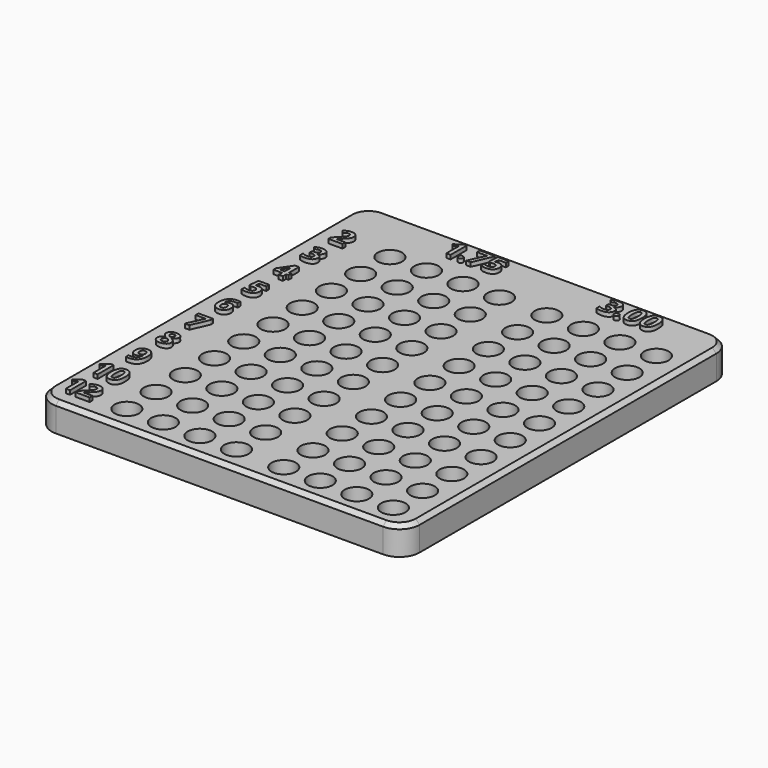
from build123d import *

# Parameters (mm, degrees)
F0_W         = 90.6357094646
F0_H         = 101.3200525194
F0_R         = 3
F1_DEPTH     = 7
F2_TEXT_SIZE = 6.9444444444
F3_DEPTH     = 1
F4_R         = 5
F5_SIZE      = 1


# Not quite as in the source:
# - Text() gives the source's letters only with a copy of the font that has no kerning and outlines rounded to 1/6400 em; it was checked with that copy


with BuildPart() as f1:
    # F0 (on Top) → F1 (new body)
    with BuildSketch(Plane.XY):
        with Locations((-1.2712031603, -23.1389431283)):
            Rectangle(F0_W, F0_H)
        with Locations((-28.8994200528, -67.7876200386)):
            Circle(F0_R, mode=Mode.SUBTRACT)
        with Locations((-28.8994200528, -58.7876200386)):
            Circle(F0_R, mode=Mode.SUBTRACT)
        with Locations((-28.8994200528, -49.7876200386)):
            Circle(F0_R, mode=Mode.SUBTRACT)
        with Locations((-19.8994200528, -67.7876200386)):
            Circle(F0_R, mode=Mode.SUBTRACT)
        with Locations((-10.8994200528, -67.7876200386)):
            Circle(F0_R, mode=Mode.SUBTRACT)
        with Locations((-1.8994200528, -67.7876200386)):
            Circle(F0_R, mode=Mode.SUBTRACT)
        with Locations((-19.8994200528, -58.7876200386)):
            Circle(F0_R, mode=Mode.SUBTRACT)
        with Locations((-19.8994200528, -49.7876200386)):
            Circle(F0_R, mode=Mode.SUBTRACT)
        with Locations((-10.8994200528, -58.7876200386)):
            Circle(F0_R, mode=Mode.SUBTRACT)
        with Locations((-1.8994200528, -58.7876200386)):
            Circle(F0_R, mode=Mode.SUBTRACT)
        with Locations((-10.8994200528, -49.7876200386)):
            Circle(F0_R, mode=Mode.SUBTRACT)
        with Locations((-1.8994200528, -49.7876200386)):
            Circle(F0_R, mode=Mode.SUBTRACT)
        with Locations((-28.8994200528, -40.7876200386)):
            Circle(F0_R, mode=Mode.SUBTRACT)
        with Locations((-28.8994200528, -31.7876200386)):
            Circle(F0_R, mode=Mode.SUBTRACT)
        with Locations((-19.8994200528, -40.7876200386)):
            Circle(F0_R, mode=Mode.SUBTRACT)
        with Locations((-10.8994200528, -40.7876200386)):
            Circle(F0_R, mode=Mode.SUBTRACT)
        with Locations((-1.8994200528, -40.7876200386)):
            Circle(F0_R, mode=Mode.SUBTRACT)
        with Locations((-19.8994200528, -31.7876200386)):
            Circle(F0_R, mode=Mode.SUBTRACT)
        with Locations((-10.8994200528, -31.7876200386)):
            Circle(F0_R, mode=Mode.SUBTRACT)
        with Locations((-1.8994200528, -31.7876200386)):
            Circle(F0_R, mode=Mode.SUBTRACT)
        with Locations((9.8412055522, -67.8979342282)):
            Circle(F0_R, mode=Mode.SUBTRACT)
        with Locations((18.8412055522, -67.8979342282)):
            Circle(F0_R, mode=Mode.SUBTRACT)
        with Locations((9.8412055522, -58.8979342282)):
            Circle(F0_R, mode=Mode.SUBTRACT)
        with Locations((9.8412055522, -49.8979342282)):
            Circle(F0_R, mode=Mode.SUBTRACT)
        with Locations((18.8412055522, -58.8979342282)):
            Circle(F0_R, mode=Mode.SUBTRACT)
        with Locations((18.8412055522, -49.8979342282)):
            Circle(F0_R, mode=Mode.SUBTRACT)
        with Locations((27.8412055522, -67.8979342282)):
            Circle(F0_R, mode=Mode.SUBTRACT)
        with Locations((36.8412055522, -67.8979342282)):
            Circle(F0_R, mode=Mode.SUBTRACT)
        with Locations((27.8412055522, -58.8979342282)):
            Circle(F0_R, mode=Mode.SUBTRACT)
        with Locations((27.8412055522, -49.8979342282)):
            Circle(F0_R, mode=Mode.SUBTRACT)
        with Locations((36.8412055522, -58.8979342282)):
            Circle(F0_R, mode=Mode.SUBTRACT)
        with Locations((36.8412055522, -49.8979342282)):
            Circle(F0_R, mode=Mode.SUBTRACT)
        with Locations((9.8412055522, -40.8979342282)):
            Circle(F0_R, mode=Mode.SUBTRACT)
        with Locations((18.8412055522, -40.8979342282)):
            Circle(F0_R, mode=Mode.SUBTRACT)
        with Locations((9.8412055522, -31.8979342282)):
            Circle(F0_R, mode=Mode.SUBTRACT)
        with Locations((18.8412055522, -31.8979342282)):
            Circle(F0_R, mode=Mode.SUBTRACT)
        with Locations((27.8412055522, -40.8979342282)):
            Circle(F0_R, mode=Mode.SUBTRACT)
        with Locations((36.8412055522, -40.8979342282)):
            Circle(F0_R, mode=Mode.SUBTRACT)
        with Locations((27.8412055522, -31.8979342282)):
            Circle(F0_R, mode=Mode.SUBTRACT)
        with Locations((36.8412055522, -31.8979342282)):
            Circle(F0_R, mode=Mode.SUBTRACT)
        with Locations((-28.8994200528, -22.7876200386)):
            Circle(F0_R, mode=Mode.SUBTRACT)
        with Locations((-28.8994200528, -13.7876200386)):
            Circle(F0_R, mode=Mode.SUBTRACT)
        with Locations((-28.8994200528, -4.7876200386)):
            Circle(F0_R, mode=Mode.SUBTRACT)
        with Locations((-19.8994200528, -22.7876200386)):
            Circle(F0_R, mode=Mode.SUBTRACT)
        with Locations((-19.8994200528, -13.7876200386)):
            Circle(F0_R, mode=Mode.SUBTRACT)
        with Locations((-10.8994200528, -22.7876200386)):
            Circle(F0_R, mode=Mode.SUBTRACT)
        with Locations((-1.8994200528, -22.7876200386)):
            Circle(F0_R, mode=Mode.SUBTRACT)
        with Locations((-10.8994200528, -13.7876200386)):
            Circle(F0_R, mode=Mode.SUBTRACT)
        with Locations((-1.8994200528, -13.7876200386)):
            Circle(F0_R, mode=Mode.SUBTRACT)
        with Locations((-19.8994200528, -4.7876200386)):
            Circle(F0_R, mode=Mode.SUBTRACT)
        with Locations((-10.8994200528, -4.7876200386)):
            Circle(F0_R, mode=Mode.SUBTRACT)
        with Locations((-1.8994200528, -4.7876200386)):
            Circle(F0_R, mode=Mode.SUBTRACT)
        with Locations((-28.8994200528, 4.2123799614)):
            Circle(F0_R, mode=Mode.SUBTRACT)
        with Locations((-28.8994200528, 13.2123799614)):
            Circle(F0_R, mode=Mode.SUBTRACT)
        with Locations((-19.8994200528, 4.2123799614)):
            Circle(F0_R, mode=Mode.SUBTRACT)
        with Locations((-19.8994200528, 13.2123799614)):
            Circle(F0_R, mode=Mode.SUBTRACT)
        with Locations((-10.8994200528, 4.2123799614)):
            Circle(F0_R, mode=Mode.SUBTRACT)
        with Locations((-1.8994200528, 4.2123799614)):
            Circle(F0_R, mode=Mode.SUBTRACT)
        with Locations((-10.8994200528, 13.2123799614)):
            Circle(F0_R, mode=Mode.SUBTRACT)
        with Locations((-1.8994200528, 13.2123799614)):
            Circle(F0_R, mode=Mode.SUBTRACT)
        with Locations((9.8412055522, -22.8979342282)):
            Circle(F0_R, mode=Mode.SUBTRACT)
        with Locations((9.8412055522, -13.8979342282)):
            Circle(F0_R, mode=Mode.SUBTRACT)
        with Locations((18.8412055522, -22.8979342282)):
            Circle(F0_R, mode=Mode.SUBTRACT)
        with Locations((18.8412055522, -13.8979342282)):
            Circle(F0_R, mode=Mode.SUBTRACT)
        with Locations((9.8412055522, -4.8979342282)):
            Circle(F0_R, mode=Mode.SUBTRACT)
        with Locations((18.8412055522, -4.8979342282)):
            Circle(F0_R, mode=Mode.SUBTRACT)
        with Locations((27.8412055522, -22.8979342282)):
            Circle(F0_R, mode=Mode.SUBTRACT)
        with Locations((27.8412055522, -13.8979342282)):
            Circle(F0_R, mode=Mode.SUBTRACT)
        with Locations((36.8412055522, -22.8979342282)):
            Circle(F0_R, mode=Mode.SUBTRACT)
        with Locations((36.8412055522, -13.8979342282)):
            Circle(F0_R, mode=Mode.SUBTRACT)
        with Locations((27.8412055522, -4.8979342282)):
            Circle(F0_R, mode=Mode.SUBTRACT)
        with Locations((36.8412055522, -4.8979342282)):
            Circle(F0_R, mode=Mode.SUBTRACT)
        with Locations((9.8412055522, 4.1020657718)):
            Circle(F0_R, mode=Mode.SUBTRACT)
        with Locations((9.8412055522, 13.1020657718)):
            Circle(F0_R, mode=Mode.SUBTRACT)
        with Locations((18.8412055522, 4.1020657718)):
            Circle(F0_R, mode=Mode.SUBTRACT)
        with Locations((18.8412055522, 13.1020657718)):
            Circle(F0_R, mode=Mode.SUBTRACT)
        with Locations((27.8412055522, 4.1020657718)):
            Circle(F0_R, mode=Mode.SUBTRACT)
        with Locations((27.8412055522, 13.1020657718)):
            Circle(F0_R, mode=Mode.SUBTRACT)
        with Locations((36.8412055522, 4.1020657718)):
            Circle(F0_R, mode=Mode.SUBTRACT)
        with Locations((36.8412055522, 13.1020657718)):
            Circle(F0_R, mode=Mode.SUBTRACT)
    extrude(amount=F1_DEPTH)

    # F4
    f4_edges = [f1.edges().sort_by_distance(p)[0] for p in [
        (-46.589058, -73.798969, 3.5),
        (44.046652, -73.798969, 3.5),
        (44.046652, 27.521083, 3.5),
        (-46.589058, 27.521083, 3.5),
    ]]
    fillet(f4_edges, radius=F4_R)

    # F5
    f5_edges = [f1.edges().sort_by_distance(p)[0] for p in [
        (-1.271203, 27.521083, 7),
    ]]
    chamfer(f5_edges, length=F5_SIZE)


with BuildPart() as f3:
    # F2 (on face) → F3 (new body)
    with BuildSketch(Plane.XY.offset(7)):
        with Locations((-22.031646253, 19.7390108928)):
            Text('1.75', F2_TEXT_SIZE, font='Open Sans', font_style=FontStyle.BOLD, text_align=(TextAlign.LEFT, TextAlign.BOTTOM))
        with Locations((16.3764719525, 19.7390108928)):
            Text('3.00', F2_TEXT_SIZE, font='Open Sans', font_style=FontStyle.BOLD, text_align=(TextAlign.LEFT, TextAlign.BOTTOM))
        with Locations((-41.9802677466, 10.2739119902)):
            Text('2', F2_TEXT_SIZE, font='Open Sans', font_style=FontStyle.BOLD, text_align=(TextAlign.LEFT, TextAlign.BOTTOM))
        with Locations((-41.9563962188, 1.3585933484)):
            Text('3', F2_TEXT_SIZE, font='Open Sans', font_style=FontStyle.BOLD, text_align=(TextAlign.LEFT, TextAlign.BOTTOM))
        with Locations((-42.036148823, -7.3902534787)):
            Text('4', F2_TEXT_SIZE, font='Open Sans', font_style=FontStyle.BOLD, text_align=(TextAlign.LEFT, TextAlign.BOTTOM))
        with Locations((-41.9346948299, -16.7467733845)):
            Text('5', F2_TEXT_SIZE, font='Open Sans', font_style=FontStyle.BOLD, text_align=(TextAlign.LEFT, TextAlign.BOTTOM))
        with Locations((-41.9802677466, -25.7000755519)):
            Text('6', F2_TEXT_SIZE, font='Open Sans', font_style=FontStyle.BOLD, text_align=(TextAlign.LEFT, TextAlign.BOTTOM))
        with Locations((-41.9802677466, -34.5483180135)):
            Text('7', F2_TEXT_SIZE, font='Open Sans', font_style=FontStyle.BOLD, text_align=(TextAlign.LEFT, TextAlign.BOTTOM))
        with Locations((-41.9699595869, -43.6492785811)):
            Text('8', F2_TEXT_SIZE, font='Open Sans', font_style=FontStyle.BOLD, text_align=(TextAlign.LEFT, TextAlign.BOTTOM))
        with Locations((-41.9699595869, -52.4123348296)):
            Text('9', F2_TEXT_SIZE, font='Open Sans', font_style=FontStyle.BOLD, text_align=(TextAlign.LEFT, TextAlign.BOTTOM))
        with Locations((-43.9485837188, -61.558727175)):
            Text('10', F2_TEXT_SIZE, font='Open Sans', font_style=FontStyle.BOLD, text_align=(TextAlign.LEFT, TextAlign.BOTTOM))
        with Locations((-43.9621470869, -70.0341304764)):
            Text('12', F2_TEXT_SIZE, font='Open Sans', font_style=FontStyle.BOLD, text_align=(TextAlign.LEFT, TextAlign.BOTTOM))
    extrude(amount=F3_DEPTH)


solid = Compound([f1.part, f3.part])
